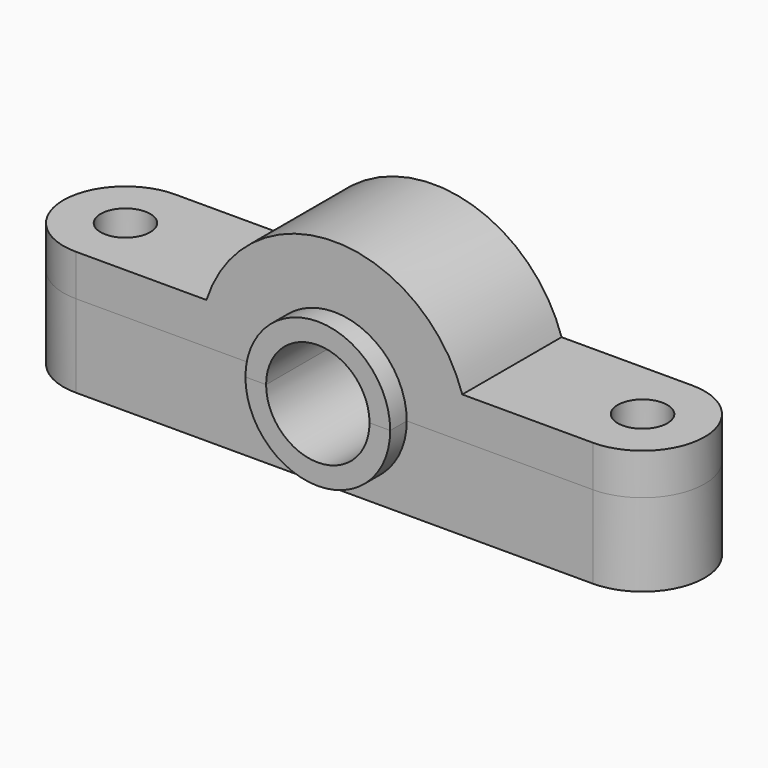
from build123d import *

# Parameters (mm, degrees)
F2_DEPTH = 21.5
F3_DEPTH = 23.9
F1_R     = 6
F4_DEPTH = 69.6
F5_DEPTH = 20
F6_DEPTH = 20


with BuildPart() as f2:
    # F0 (on Front) → F2 (new body, symmetric)
    with BuildSketch(Plane.XZ):
        with BuildLine():
            Line((-116.4417862892, 0), (0, 0))
            Line((0, 0), (116.4417862892, 0))
            Line((116.4417862892, 0), (116.4417862892, 20))
            Line((116.4417862892, 20), (17.5, 20))
            ThreePointArc((17.5, 20), (0, 2.5), (-17.5, 20))
            Line((-17.5, 20), (-116.4417862892, 20))
            Line((-116.4417862892, 20), (-116.4417862892, 0))
        make_face()
    extrude(amount=F2_DEPTH, both=True)


with BuildPart() as f3:
    # F0 (on Front) → F3 (new body, symmetric)
    with BuildSketch(Plane.XZ):
        with BuildLine():
            Line((-116.4417862892, 30), (-116.4417862892, 20))
            Line((-116.4417862892, 20), (-17.5, 20))
            ThreePointArc((-17.5, 20), (0, 37.5), (17.5, 20))
            Line((17.5, 20), (116.4417862892, 20))
            Line((116.4417862892, 20), (116.4417862892, 30))
            Line((116.4417862892, 30), (30.9232921921, 30))
            ThreePointArc((30.9232921921, 30), (0, 52.5), (-30.9232921921, 30))
            Line((-30.9232921921, 30), (-116.4417862892, 30))
        make_face()
    extrude(amount=F3_DEPTH, both=True)


with BuildPart() as f4_tool:
    # F1 (on Top) → F4 (new body)
    with BuildSketch(Plane.XY):
        with BuildLine():
            Line((62.5, 15), (-62.5, 15))
            ThreePointArc((-62.5, 15), (-77.5, 0), (-62.5, -15))
            Line((-62.5, -15), (62.5, -15))
            ThreePointArc((62.5, -15), (77.5, 0), (62.5, 15))
        make_face()
        with Locations((-62.5, 0)):
            Circle(F1_R, mode=Mode.SUBTRACT)
        with Locations((62.5, 0)):
            Circle(F1_R, mode=Mode.SUBTRACT)
    extrude(amount=F4_DEPTH)


with BuildPart() as f2_1:
    add(f2.part)

    # F4: intersect by f4_tool
    add(f4_tool.part, mode=Mode.INTERSECT)

    # F0 (on Front) → F5 (join, symmetric)
    with BuildSketch(Plane.XZ):
        with BuildLine():
            Line((-12.5, 20), (-17.5, 20))
            ThreePointArc((-17.5, 20), (0, 2.5), (17.5, 20))
            Line((17.5, 20), (12.5, 20))
            ThreePointArc((12.5, 20), (0, 7.5), (-12.5, 20))
        make_face()
    extrude(amount=F5_DEPTH, both=True)


with BuildPart() as f3_1:
    add(f3.part)

    # F4: intersect by f4_tool
    add(f4_tool.part, mode=Mode.INTERSECT)

    # F0 (on Front) → F6 (join, symmetric)
    with BuildSketch(Plane.XZ):
        with BuildLine():
            ThreePointArc((17.5, 20), (0, 37.5), (-17.5, 20))
            Line((-17.5, 20), (-12.5, 20))
            ThreePointArc((-12.5, 20), (0, 32.5), (12.5, 20))
            Line((12.5, 20), (17.5, 20))
        make_face()
    extrude(amount=F6_DEPTH, both=True)


solid = Compound([f2_1.part, f3_1.part])
